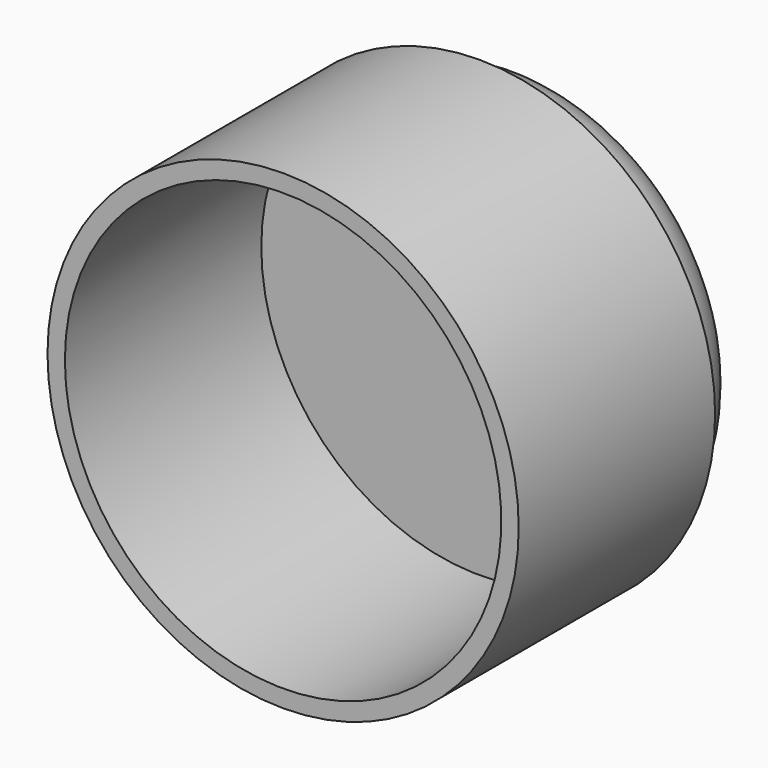
from build123d import *

# Parameters (mm, degrees)
F0_R     = 17.275
F1_DEPTH = 18
F3_D     = 32
F4_R     = 16.275
F5_DEPTH = 5
F6_R     = 4.99999


# Not quite as in the source:
# - a fillet or chamfer is up to 0.001 mm smaller than in the source, because OpenCascade refuses the exact size


with BuildPart() as f1:
    # F0 (on Front) → F1 (new body)
    with BuildSketch(Plane.XZ):
        Circle(F0_R)
    extrude(amount=F1_DEPTH)

    # F3 (through all)
    with Locations(Plane(origin=(0, 0, 0), x_dir=(1, 0, 0), z_dir=(0, 1, 0))):
        with Locations((0, 0)):
            Hole(F3_D / 2)

    # F4 (on Front) → F5 (join)
    with BuildSketch(Plane.XZ):
        Circle(F4_R)
    extrude(amount=-F5_DEPTH)

    # F6 (radius 5 in the source; OpenCascade refuses exactly that, so slightly less here)
    f6_edges = [f1.edges().sort_by_distance(p)[0] for p in [
        (-16.275, 5, 0),
    ]]
    fillet(f6_edges, radius=F6_R)


solid = f1.part
